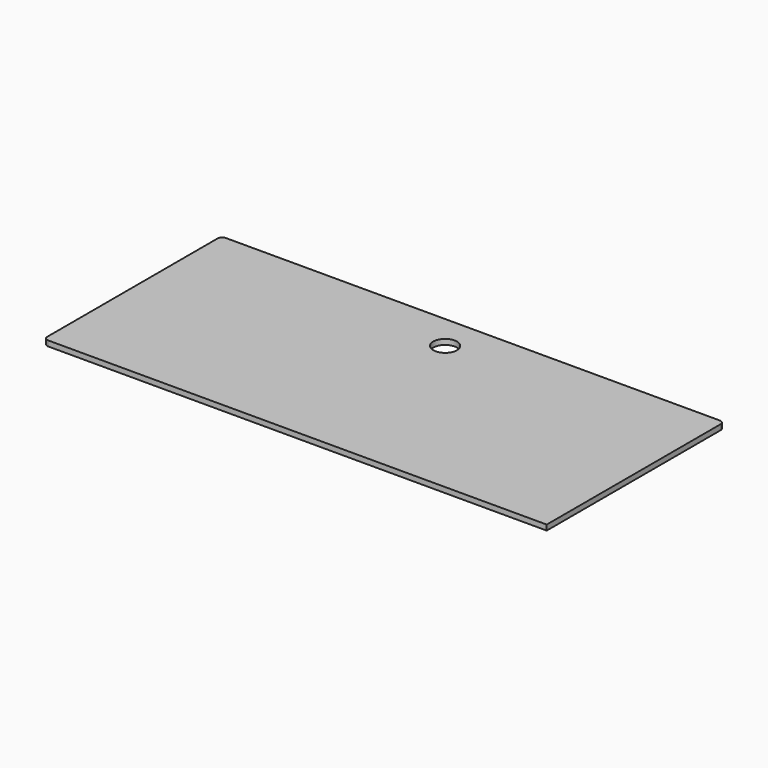
from build123d import *

# Parameters (mm, degrees)
F1_DEPTH = 18
F2_R     = 15
F4_D     = 8
F4_DEPTH = 15
F4_TIP   = 2.4034424761
F6_DEPTH = 18


# Not quite as in the source:
# - a feature names something its author has since deleted; it is built from what else it names


with BuildPart() as f1:
    # F0 (on Top) → F1 (new body)
    with BuildSketch(Plane.XY):
        Polygon((1700, 0), (0, 0), (0, -750), (1690, -750), (1700, -750), align=None)
    extrude(amount=F1_DEPTH)

    # F2
    f2_edges = [f1.edges().sort_by_distance(p)[0] for p in [
        (0, -750, 9),
        (0, 0, 9),
        (1700, 0, 9),
    ]]
    fillet(f2_edges, radius=F2_R)

    # F4
    with Locations(Plane(origin=(0, 0, 0), x_dir=(1, 0, 0), z_dir=(0, 0, -1))):
        with Locations((136.6116523517, 286.6116523517), (100, 250), (100, 375), (136.6116523517, 463.3883476483), (100, 500), (313.3883476483, 463.3883476483), (350, 375), (313.3883476483, 286.6116523517), (1200, 150), (1450, 150), (1589.5405845398, 110.4594154602), (1600, 250), (1450, 375), (1200, 375), (1417.1572875254, 467.1572875254), (1600, 500), (1593.933982822, 643.933982822), (1450, 650), (1200, 650), (1412.7638892432, 287.2361107568)):
            Hole(F4_D / 2, depth=F4_DEPTH)
            with Locations((0, 0, -(F4_DEPTH + F4_TIP / 2))):  # 118° drill point
                Cone(0, F4_D / 2, F4_TIP, mode=Mode.SUBTRACT)

    # F5 (on face) → F6 (cut)
    with BuildSketch(Plane(origin=(0, 0, 0), x_dir=(1, 0, 0), z_dir=(0, 0, -1))):
        with BuildLine():
            ThreePointArc((851.6666666667, 79.9826370047), (880.4880927062, 91.3965751745), (892.5, 119.973955507))
            ThreePointArc((892.5, 119.973955507), (824.5119072938, 148.5513358395), (851.6666666667, 79.9826370047))
        make_face()
    extrude(amount=-F6_DEPTH, mode=Mode.SUBTRACT)


solid = f1.part
